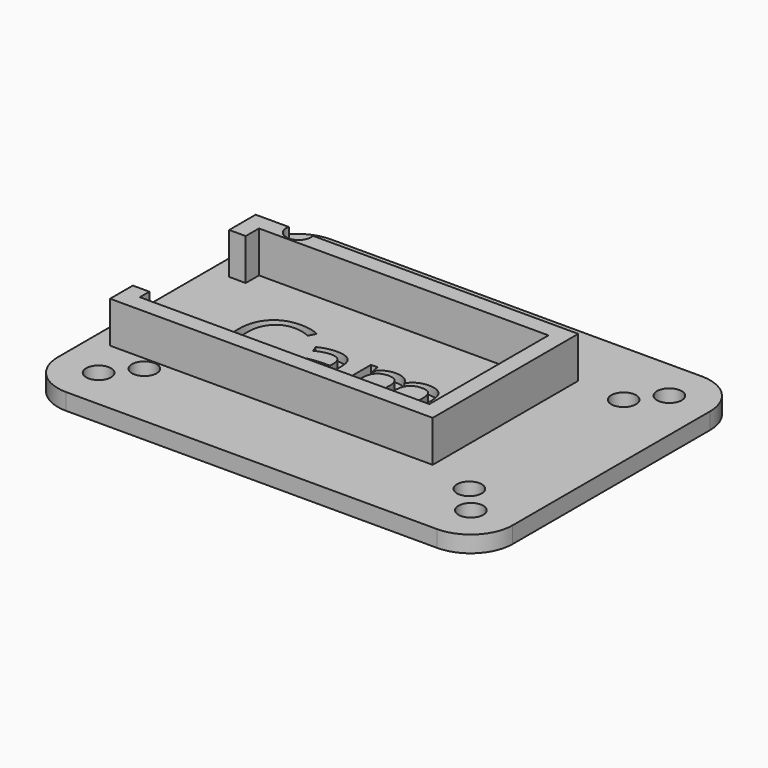
from build123d import *

# Parameters (mm, degrees)
F0_W         = 55
F0_H         = 40
F1_DEPTH     = 2
F3_R         = 5.08
F4_R         = 5.08
F5_R         = 5.08
F6_R         = 5.08
F8_TEXT_SIZE = 11.8391950511
F9_DEPTH     = 1
F11_DEPTH    = 5
F12_R        = 1.5
F13_DEPTH    = 12.7


# Not quite as in the source:
# - Text() gives the source's letters only with a copy of the font that has no kerning and outlines rounded to 1/6400 em; it was checked with that copy


with BuildPart() as f1:
    # F0 (on Top) → F1 (new body)
    with BuildSketch(Plane.XY):
        with Locations((27.5, 20)):
            Rectangle(F0_W, F0_H)
    extrude(amount=F1_DEPTH)

    # F3
    f3_edges = [f1.edges().sort_by_distance(p)[0] for p in [
        (55, 0, 1),
    ]]
    fillet(f3_edges, radius=F3_R)

    # F4
    f4_edges = [f1.edges().sort_by_distance(p)[0] for p in [
        (55, 40, 1),
    ]]
    fillet(f4_edges, radius=F4_R)

    # F5
    f5_edges = [f1.edges().sort_by_distance(p)[0] for p in [
        (0, 40, 1),
    ]]
    fillet(f5_edges, radius=F5_R)

    # F6
    f6_edges = [f1.edges().sort_by_distance(p)[0] for p in [
        (0, 0, 1),
    ]]
    fillet(f6_edges, radius=F6_R)

    # F8 (on offset) → F9 (cut)
    with BuildSketch(Plane.XY.offset(2)):
        with Locations((8.9907050133, 16)):
            Text('Cam', F8_TEXT_SIZE, font='Open Sans', text_align=(TextAlign.LEFT, TextAlign.BOTTOM))
    extrude(amount=-F9_DEPTH, mode=Mode.SUBTRACT)

    # F10 (on offset) → F11 (join)
    with BuildSketch(Plane.XY.offset(2)):
        Polygon((4.3826700747, 28), (4.3826700747, 30), (39.3826700747, 30), (39.3826700747, 12), (4.3826700747, 12), (4.3826700747, 13.4396387637), (2.3826700747, 13.4396387637), (2.3826700747, 10), (41.3826700747, 10), (41.3826700747, 32), (2.3826700747, 32), (2.3826700747, 28), align=None)
    extrude(amount=F11_DEPTH)

    # F12 (on offset) → F13 (cut, symmetric)
    with BuildSketch(Plane.XY.offset(2)):
        with Locations((50, 5)):
            Circle(F12_R)
        with Locations((47.1494022449, 8.3385913854)):
            Circle(F12_R)
        with Locations((47.1494022449, 31.6614086146)):
            Circle(F12_R)
        with Locations((50, 35)):
            Circle(F12_R)
        with Locations((7.8505977551, 31.6614086146)):
            Circle(F12_R)
        with Locations((5, 35)):
            Circle(F12_R)
        with Locations((7.8505977551, 8.3385913854)):
            Circle(F12_R)
        with Locations((5, 5)):
            Circle(F12_R)
    extrude(amount=F13_DEPTH, both=True, mode=Mode.SUBTRACT)


solid = f1.part
